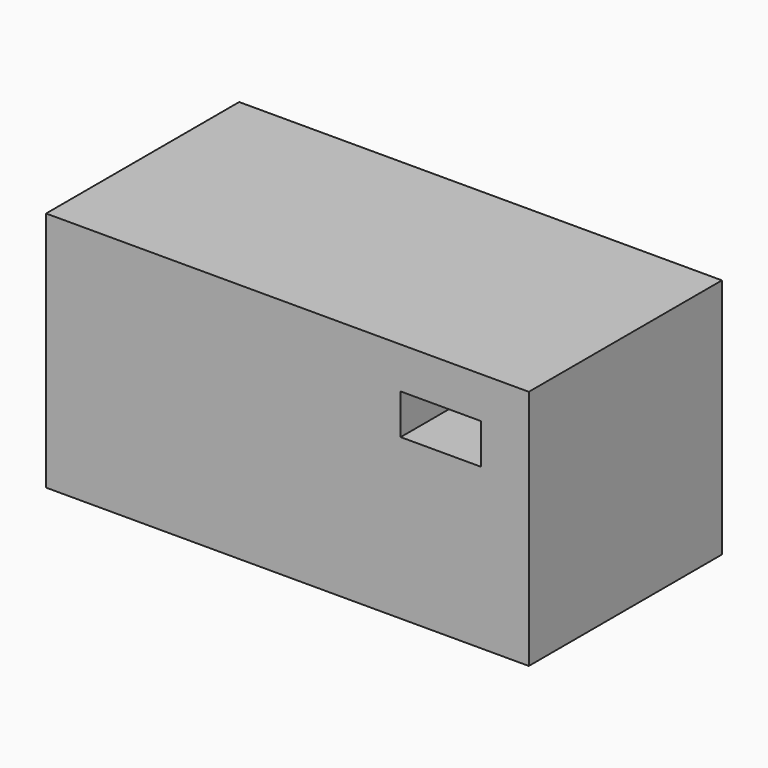
from build123d import *

# Parameters (mm, degrees)
F0_W     = 76.2
F0_H     = 38.1
F0_W_2   = 12.7
F0_H_2   = 6.35
F1_DEPTH = 38.1


# Not quite as in the source:
# - the program builds the solid bodies; features that only make, move or delete a surface that nothing else refers to are left out


with BuildPart() as f1:
    # F0 (on Front) → F1 (new body)
    with BuildSketch(Plane.XZ):
        with Locations((-24.3708645046, 23.7796551056)):
            Rectangle(F0_W, F0_H)
        with Locations((-0.1532746643, 33.1294818699)):
            Rectangle(F0_W_2, F0_H_2, mode=Mode.SUBTRACT)
    extrude(amount=F1_DEPTH)


solid = f1.part
